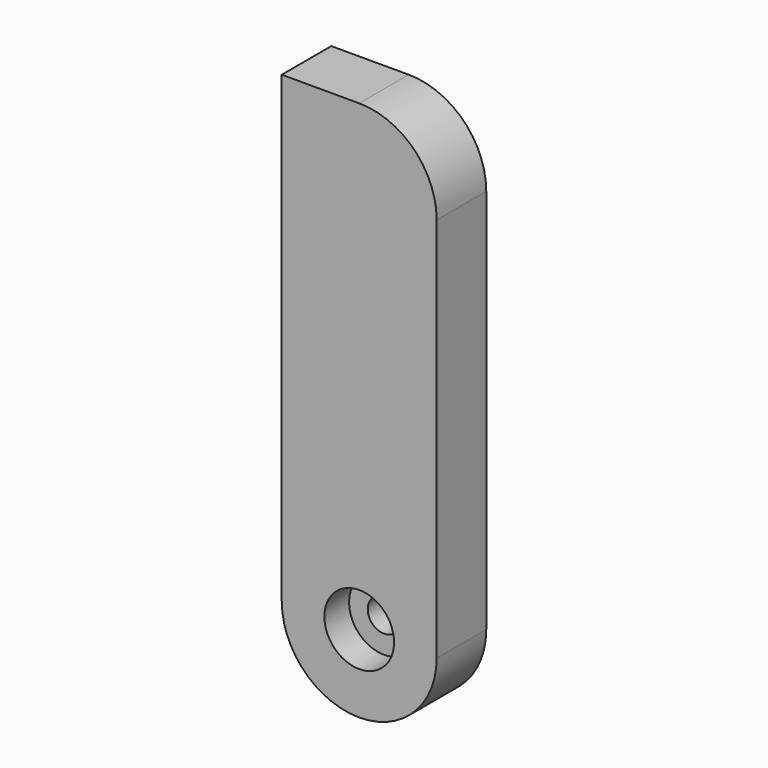
from build123d import *

# Parameters (mm, degrees)
F0_W     = 10
F0_H     = 34.9
F1_DEPTH = 4
F2_R     = 5
F3_R     = 4.99999
F4_R     = 2.25
F4_R_2   = 1.05
F5_DEPTH = 2
F6_DEPTH = 5


# Not quite as in the source:
# - a fillet or chamfer is up to 0.001 mm smaller than in the source, because OpenCascade refuses the exact size


with BuildPart() as f1:
    # F0 (on Front) → F1 (new body)
    with BuildSketch(Plane.XZ):
        Rectangle(F0_W, F0_H)
    extrude(amount=F1_DEPTH)

    # F2
    f2_edges = [f1.edges().sort_by_distance(p)[0] for p in [
        (5, -2, 17.45),
    ]]
    fillet(f2_edges, radius=F2_R)

    # F3 (radius 5 in the source; OpenCascade refuses exactly that, so slightly less here)
    f3_edges = [f1.edges().sort_by_distance(p)[0] for p in [
        (5, -2, -17.45),
        (-5, -2, -17.45),
    ]]
    fillet(f3_edges, radius=F3_R)

    # F4 (on face) → F5 (cut)
    with BuildSketch(Plane.XZ.offset(4)):
        with Locations((0, -12.45)):
            Circle(F4_R)
        with Locations((0, -12.45)):
            Circle(F4_R_2, mode=Mode.SUBTRACT)
    extrude(amount=-F5_DEPTH, mode=Mode.SUBTRACT)

    # F6 (cut): a face of the model
    f6_faces = [f1.faces().sort_by_distance(p)[0] for p in [
        (0, -4, -12.45),
    ]]
    extrude(f6_faces, amount=-F6_DEPTH, mode=Mode.SUBTRACT)


solid = f1.part
